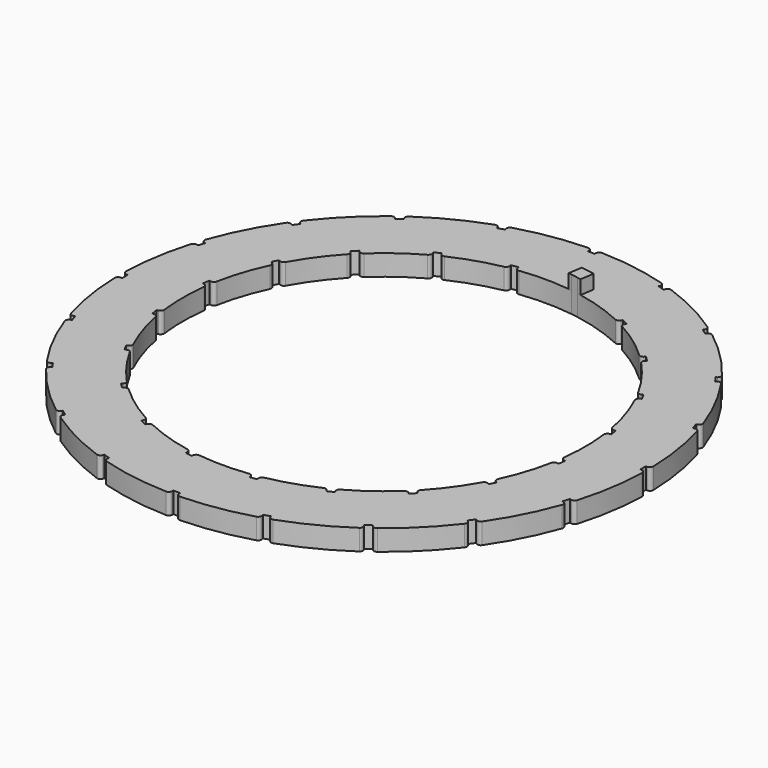
from build123d import *
from build123d import SkipClean  # not in build123d's __all__

# Parameters (mm, degrees)
F0_R     = 19
F0_R_2   = 14.5
F1_DEPTH = 1.5
F3_DEPTH = 1.501
F5_DEPTH = 1.501
F7_DEPTH = 2.5
F9_DEPTH = 1
F10_R    = 0.25
F11_R    = 0.25


with BuildPart() as f1:
    # F0 (on Top) → F1 (new body)
    with BuildSketch(Plane.XY):
        Circle(F0_R)
        Circle(F0_R_2, mode=Mode.SUBTRACT)
    extrude(amount=F1_DEPTH)

    # F2 (on face) → F3 (cut, through all)
    with BuildSketch(Plane.XY.offset(1.5)):
        with BuildLine():
            ThreePointArc((0.25, 18.998355192), (0, 19), (-0.25, 18.998355192))
            Line((-0.25, 18.998355192), (-0.25, 18.648355192))
            Line((-0.25, 18.648355192), (0.25, 18.648355192))
            Line((0.25, 18.648355192), (0.25, 18.998355192))
        make_face()
        with BuildLine():
            ThreePointArc((-5.6330504904, 18.1457637528), (-5.8713228931, 18.0700738096), (-6.1085787486, 17.9912552556))
            Line((-6.1085787486, 17.9912552556), (-6.0004228005, 17.6583854749))
            Line((-6.0004228005, 17.6583854749), (-5.5248945424, 17.8128939721))
            Line((-5.5248945424, 17.8128939721), (-5.6330504904, 18.1457637528))
        make_face()
        with BuildLine():
            ThreePointArc((-10.9646987511, 15.5169385285), (-11.1679197936, 15.3713228931), (-11.3692072482, 15.2230459024))
            Line((-11.3692072482, 15.2230459024), (-11.1634824099, 14.9398899544))
            Line((-11.1634824099, 14.9398899544), (-10.7589739128, 15.2337825805))
            Line((-10.7589739128, 15.2337825805), (-10.9646987511, 15.5169385285))
        make_face()
        with BuildLine():
            ThreePointArc((-15.2230459024, 11.3692072482), (-15.3713228931, 11.1679197936), (-15.5169385285, 10.9646987511))
            Line((-15.5169385285, 10.9646987511), (-15.2337825805, 10.7589739128))
            Line((-15.2337825805, 10.7589739128), (-14.9398899544, 11.1634824099))
            Line((-14.9398899544, 11.1634824099), (-15.2230459024, 11.3692072482))
        make_face()
        with BuildLine():
            ThreePointArc((-17.9912552556, 6.1085787486), (-18.0700738096, 5.8713228931), (-18.1457637528, 5.6330504904))
            Line((-18.1457637528, 5.6330504904), (-17.8128939721, 5.5248945424))
            Line((-17.8128939721, 5.5248945424), (-17.6583854749, 6.0004228005))
            Line((-17.6583854749, 6.0004228005), (-17.9912552556, 6.1085787486))
        make_face()
        with BuildLine():
            ThreePointArc((-18.998355192, 0.25), (-19, 0), (-18.998355192, -0.25))
            Line((-18.998355192, -0.25), (-18.648355192, -0.25))
            Line((-18.648355192, -0.25), (-18.648355192, 0.25))
            Line((-18.648355192, 0.25), (-18.998355192, 0.25))
        make_face()
        with BuildLine():
            ThreePointArc((-18.1457637528, -5.6330504904), (-18.0700738096, -5.8713228931), (-17.9912552556, -6.1085787486))
            Line((-17.9912552556, -6.1085787486), (-17.6583854749, -6.0004228005))
            Line((-17.6583854749, -6.0004228005), (-17.8128939721, -5.5248945424))
            Line((-17.8128939721, -5.5248945424), (-18.1457637528, -5.6330504904))
        make_face()
        with BuildLine():
            ThreePointArc((-15.5169385285, -10.9646987511), (-15.3713228931, -11.1679197936), (-15.2230459024, -11.3692072482))
            Line((-15.2230459024, -11.3692072482), (-14.9398899544, -11.1634824099))
            Line((-14.9398899544, -11.1634824099), (-15.2337825805, -10.7589739128))
            Line((-15.2337825805, -10.7589739128), (-15.5169385285, -10.9646987511))
        make_face()
        with BuildLine():
            ThreePointArc((-11.3692072482, -15.2230459024), (-11.1679197936, -15.3713228931), (-10.9646987511, -15.5169385285))
            Line((-10.9646987511, -15.5169385285), (-10.7589739128, -15.2337825805))
            Line((-10.7589739128, -15.2337825805), (-11.1634824099, -14.9398899544))
            Line((-11.1634824099, -14.9398899544), (-11.3692072482, -15.2230459024))
        make_face()
        with BuildLine():
            ThreePointArc((-6.1085787486, -17.9912552556), (-5.8713228931, -18.0700738096), (-5.6330504904, -18.1457637528))
            Line((-5.6330504904, -18.1457637528), (-5.5248945424, -17.8128939721))
            Line((-5.5248945424, -17.8128939721), (-6.0004228005, -17.6583854749))
            Line((-6.0004228005, -17.6583854749), (-6.1085787486, -17.9912552556))
        make_face()
        with BuildLine():
            ThreePointArc((-0.25, -18.998355192), (0, -19), (0.25, -18.998355192))
            Line((0.25, -18.998355192), (0.25, -18.648355192))
            Line((0.25, -18.648355192), (-0.25, -18.648355192))
            Line((-0.25, -18.648355192), (-0.25, -18.998355192))
        make_face()
        with BuildLine():
            ThreePointArc((5.6330504904, -18.1457637528), (5.8713228931, -18.0700738096), (6.1085787486, -17.9912552556))
            Line((6.1085787486, -17.9912552556), (6.0004228005, -17.6583854749))
            Line((6.0004228005, -17.6583854749), (5.5248945424, -17.8128939721))
            Line((5.5248945424, -17.8128939721), (5.6330504904, -18.1457637528))
        make_face()
        with BuildLine():
            ThreePointArc((10.9646987511, -15.5169385285), (11.1679197936, -15.3713228931), (11.3692072482, -15.2230459024))
            Line((11.3692072482, -15.2230459024), (11.1634824099, -14.9398899544))
            Line((11.1634824099, -14.9398899544), (10.7589739128, -15.2337825805))
            Line((10.7589739128, -15.2337825805), (10.9646987511, -15.5169385285))
        make_face()
        with BuildLine():
            ThreePointArc((15.2230459024, -11.3692072482), (15.3713228931, -11.1679197936), (15.5169385285, -10.9646987511))
            Line((15.5169385285, -10.9646987511), (15.2337825805, -10.7589739128))
            Line((15.2337825805, -10.7589739128), (14.9398899544, -11.1634824099))
            Line((14.9398899544, -11.1634824099), (15.2230459024, -11.3692072482))
        make_face()
        with BuildLine():
            ThreePointArc((17.9912552556, -6.1085787486), (18.0700738096, -5.8713228931), (18.1457637528, -5.6330504904))
            Line((18.1457637528, -5.6330504904), (17.8128939721, -5.5248945424))
            Line((17.8128939721, -5.5248945424), (17.6583854749, -6.0004228005))
            Line((17.6583854749, -6.0004228005), (17.9912552556, -6.1085787486))
        make_face()
        with BuildLine():
            ThreePointArc((18.998355192, -0.25), (19, 0), (18.998355192, 0.25))
            Line((18.998355192, 0.25), (18.648355192, 0.25))
            Line((18.648355192, 0.25), (18.648355192, -0.25))
            Line((18.648355192, -0.25), (18.998355192, -0.25))
        make_face()
        with BuildLine():
            ThreePointArc((18.1457637528, 5.6330504904), (18.0700738096, 5.8713228931), (17.9912552556, 6.1085787486))
            Line((17.9912552556, 6.1085787486), (17.6583854749, 6.0004228005))
            Line((17.6583854749, 6.0004228005), (17.8128939721, 5.5248945424))
            Line((17.8128939721, 5.5248945424), (18.1457637528, 5.6330504904))
        make_face()
        with BuildLine():
            ThreePointArc((15.5169385285, 10.9646987511), (15.3713228931, 11.1679197936), (15.2230459024, 11.3692072482))
            Line((15.2230459024, 11.3692072482), (14.9398899544, 11.1634824099))
            Line((14.9398899544, 11.1634824099), (15.2337825805, 10.7589739128))
            Line((15.2337825805, 10.7589739128), (15.5169385285, 10.9646987511))
        make_face()
        with BuildLine():
            ThreePointArc((11.3692072482, 15.2230459024), (11.1679197936, 15.3713228931), (10.9646987511, 15.5169385285))
            Line((10.9646987511, 15.5169385285), (10.7589739128, 15.2337825805))
            Line((10.7589739128, 15.2337825805), (11.1634824099, 14.9398899544))
            Line((11.1634824099, 14.9398899544), (11.3692072482, 15.2230459024))
        make_face()
        with BuildLine():
            ThreePointArc((6.1085787486, 17.9912552556), (5.8713228931, 18.0700738096), (5.6330504904, 18.1457637528))
            Line((5.6330504904, 18.1457637528), (5.5248945424, 17.8128939721))
            Line((5.5248945424, 17.8128939721), (6.0004228005, 17.6583854749))
            Line((6.0004228005, 17.6583854749), (6.1085787486, 17.9912552556))
        make_face()
    extrude(amount=-F3_DEPTH, mode=Mode.SUBTRACT)

    # F4 (on face) → F5 (cut, through all)
    with BuildSketch(Plane.XY.offset(1.5)):
        with BuildLine():
            Line((-2.5696367227, 14.6259344447), (-2.5148846599, 14.2802435255))
            ThreePointArc((-2.5148846599, 14.2802435255), (-2.2682997431, 14.3214809386), (-2.0210404896, 14.358460758))
            Line((-2.0210404896, 14.358460758), (-2.0757925524, 14.7041516772))
            Line((-2.0757925524, 14.7041516772), (-2.5696367227, 14.6259344447))
        make_face()
        with BuildLine():
            Line((-6.9635320517, 13.1160288439), (-6.8046353767, 12.8041765604))
            ThreePointArc((-6.8046353767, 12.8041765604), (-6.5828622462, 12.9195946007), (-6.3591321147, 13.0311718103))
            Line((-6.3591321147, 13.0311718103), (-6.5180287896, 13.3430240937))
            Line((-6.5180287896, 13.3430240937), (-6.9635320517, 13.1160288439))
        make_face()
        with BuildLine():
            Line((-10.6757883456, 10.322234955), (-10.4283009722, 10.0747475816))
            ThreePointArc((-10.4283009722, 10.0747475816), (-10.2530483272, 10.2530483272), (-10.0747475816, 10.4283009722))
            Line((-10.0747475816, 10.4283009722), (-10.322234955, 10.6757883456))
            Line((-10.322234955, 10.6757883456), (-10.6757883456, 10.322234955))
        make_face()
        with BuildLine():
            Line((-13.3430240937, 6.5180287896), (-13.0311718103, 6.3591321147))
            ThreePointArc((-13.0311718103, 6.3591321147), (-12.9195946007, 6.5828622462), (-12.8041765604, 6.8046353767))
            Line((-12.8041765604, 6.8046353767), (-13.1160288439, 6.9635320517))
            Line((-13.1160288439, 6.9635320517), (-13.3430240937, 6.5180287896))
        make_face()
        with BuildLine():
            Line((-14.7041516772, 2.0757925524), (-14.358460758, 2.0210404896))
            ThreePointArc((-14.358460758, 2.0210404896), (-14.3214809386, 2.2682997431), (-14.2802435255, 2.5148846599))
            Line((-14.2802435255, 2.5148846599), (-14.6259344447, 2.5696367227))
            Line((-14.6259344447, 2.5696367227), (-14.7041516772, 2.0757925524))
        make_face()
        with BuildLine():
            Line((-14.6259344447, -2.5696367227), (-14.2802435255, -2.5148846599))
            ThreePointArc((-14.2802435255, -2.5148846599), (-14.3214809386, -2.2682997431), (-14.358460758, -2.0210404896))
            Line((-14.358460758, -2.0210404896), (-14.7041516772, -2.0757925524))
            Line((-14.7041516772, -2.0757925524), (-14.6259344447, -2.5696367227))
        make_face()
        with BuildLine():
            Line((-13.1160288439, -6.9635320517), (-12.8041765604, -6.8046353767))
            ThreePointArc((-12.8041765604, -6.8046353767), (-12.9195946007, -6.5828622462), (-13.0311718103, -6.3591321147))
            Line((-13.0311718103, -6.3591321147), (-13.3430240937, -6.5180287896))
            Line((-13.3430240937, -6.5180287896), (-13.1160288439, -6.9635320517))
        make_face()
        with BuildLine():
            Line((-10.322234955, -10.6757883456), (-10.0747475816, -10.4283009722))
            ThreePointArc((-10.0747475816, -10.4283009722), (-10.2530483272, -10.2530483272), (-10.4283009722, -10.0747475816))
            Line((-10.4283009722, -10.0747475816), (-10.6757883456, -10.322234955))
            Line((-10.6757883456, -10.322234955), (-10.322234955, -10.6757883456))
        make_face()
        with BuildLine():
            Line((-6.5180287896, -13.3430240937), (-6.3591321147, -13.0311718103))
            ThreePointArc((-6.3591321147, -13.0311718103), (-6.5828622462, -12.9195946007), (-6.8046353767, -12.8041765604))
            Line((-6.8046353767, -12.8041765604), (-6.9635320517, -13.1160288439))
            Line((-6.9635320517, -13.1160288439), (-6.5180287896, -13.3430240937))
        make_face()
        with BuildLine():
            Line((-2.0757925524, -14.7041516772), (-2.0210404896, -14.358460758))
            ThreePointArc((-2.0210404896, -14.358460758), (-2.2682997431, -14.3214809386), (-2.5148846599, -14.2802435255))
            Line((-2.5148846599, -14.2802435255), (-2.5696367227, -14.6259344447))
            Line((-2.5696367227, -14.6259344447), (-2.0757925524, -14.7041516772))
        make_face()
        with BuildLine():
            Line((2.5696367227, -14.6259344447), (2.5148846599, -14.2802435255))
            ThreePointArc((2.5148846599, -14.2802435255), (2.2682997431, -14.3214809386), (2.0210404896, -14.358460758))
            Line((2.0210404896, -14.358460758), (2.0757925524, -14.7041516772))
            Line((2.0757925524, -14.7041516772), (2.5696367227, -14.6259344447))
        make_face()
        with BuildLine():
            Line((6.9635320517, -13.1160288439), (6.8046353767, -12.8041765604))
            ThreePointArc((6.8046353767, -12.8041765604), (6.5828622462, -12.9195946007), (6.3591321147, -13.0311718103))
            Line((6.3591321147, -13.0311718103), (6.5180287896, -13.3430240937))
            Line((6.5180287896, -13.3430240937), (6.9635320517, -13.1160288439))
        make_face()
        with BuildLine():
            Line((10.6757883456, -10.322234955), (10.4283009722, -10.0747475816))
            ThreePointArc((10.4283009722, -10.0747475816), (10.2530483272, -10.2530483272), (10.0747475816, -10.4283009722))
            Line((10.0747475816, -10.4283009722), (10.322234955, -10.6757883456))
            Line((10.322234955, -10.6757883456), (10.6757883456, -10.322234955))
        make_face()
        with BuildLine():
            Line((13.3430240937, -6.5180287896), (13.0311718103, -6.3591321147))
            ThreePointArc((13.0311718103, -6.3591321147), (12.9195946007, -6.5828622462), (12.8041765604, -6.8046353767))
            Line((12.8041765604, -6.8046353767), (13.1160288439, -6.9635320517))
            Line((13.1160288439, -6.9635320517), (13.3430240937, -6.5180287896))
        make_face()
        with BuildLine():
            Line((14.7041516772, -2.0757925524), (14.358460758, -2.0210404896))
            ThreePointArc((14.358460758, -2.0210404896), (14.3214809386, -2.2682997431), (14.2802435255, -2.5148846599))
            Line((14.2802435255, -2.5148846599), (14.6259344447, -2.5696367227))
            Line((14.6259344447, -2.5696367227), (14.7041516772, -2.0757925524))
        make_face()
        with BuildLine():
            Line((14.6259344447, 2.5696367227), (14.2802435255, 2.5148846599))
            ThreePointArc((14.2802435255, 2.5148846599), (14.3214809386, 2.2682997431), (14.358460758, 2.0210404896))
            Line((14.358460758, 2.0210404896), (14.7041516772, 2.0757925524))
            Line((14.7041516772, 2.0757925524), (14.6259344447, 2.5696367227))
        make_face()
        with BuildLine():
            Line((13.1160288439, 6.9635320517), (12.8041765604, 6.8046353767))
            ThreePointArc((12.8041765604, 6.8046353767), (12.9195946007, 6.5828622462), (13.0311718103, 6.3591321147))
            Line((13.0311718103, 6.3591321147), (13.3430240937, 6.5180287896))
            Line((13.3430240937, 6.5180287896), (13.1160288439, 6.9635320517))
        make_face()
        with BuildLine():
            Line((10.322234955, 10.6757883456), (10.0747475816, 10.4283009722))
            ThreePointArc((10.0747475816, 10.4283009722), (10.2530483272, 10.2530483272), (10.4283009722, 10.0747475816))
            Line((10.4283009722, 10.0747475816), (10.6757883456, 10.322234955))
            Line((10.6757883456, 10.322234955), (10.322234955, 10.6757883456))
        make_face()
        with BuildLine():
            Line((6.5180287896, 13.3430240937), (6.3591321147, 13.0311718103))
            ThreePointArc((6.3591321147, 13.0311718103), (6.5828622462, 12.9195946007), (6.8046353767, 12.8041765604))
            Line((6.8046353767, 12.8041765604), (6.9635320517, 13.1160288439))
            Line((6.9635320517, 13.1160288439), (6.5180287896, 13.3430240937))
        make_face()
        with BuildLine():
            Line((2.0757925524, 14.7041516772), (2.0210404896, 14.358460758))
            ThreePointArc((2.0210404896, 14.358460758), (2.2682997431, 14.3214809386), (2.5148846599, 14.2802435255))
            Line((2.5148846599, 14.2802435255), (2.5696367227, 14.6259344447))
            Line((2.5696367227, 14.6259344447), (2.0757925524, 14.7041516772))
        make_face()
    extrude(amount=-F5_DEPTH, mode=Mode.SUBTRACT)

    # F6 (on face) → F7 (join)
    with BuildSketch(Plane(origin=(0, 0, 0), x_dir=(1, 0, 0), z_dir=(0, 0, -1))):
        with BuildLine():
            Line((2.5696367227, -14.6259344447), (2.5148846599, -14.2802435255))
            ThreePointArc((2.5148846599, -14.2802435255), (2.2682997431, -14.3214809386), (2.0210404896, -14.358460758))
            Line((2.0210404896, -14.358460758), (2.0757925524, -14.7041516772))
            Line((2.0757925524, -14.7041516772), (2.5696367227, -14.6259344447))
        make_face()
    extrude(amount=-F7_DEPTH)

    # F8 (on face) → F9 (join, through all)
    with BuildSketch(Plane.XY.offset(1.5)):
        with BuildLine():
            Line((1.9295410637, 15.3788694245), (1.7731065987, 14.3911810839))
            ThreePointArc((1.7731065987, 14.3911810839), (2.2682997431, 14.3214809386), (2.7607949393, 14.2347466189))
            Line((2.7607949393, 14.2347466189), (2.9172294043, 15.2224349595))
            Line((2.9172294043, 15.2224349595), (1.9295410637, 15.3788694245))
        make_face()
    with SkipClean():  # cleaning this boolean's faces spoils the solid; the shape is the same uncleaned
        extrude(amount=F9_DEPTH)

    # F10
    f10_edges = [f1.edges().sort_by_distance(p)[0] for p in [
        (6.108579, 17.991255, 0.75),
        (5.63305, 18.145764, 0.75),
        (0.25, 18.998355, 0.75),
        (-0.25, 18.998355, 0.75),
        (-5.63305, 18.145764, 0.75),
        (-6.108579, 17.991255, 0.75),
        (10.964699, 15.516939, 0.75),
        (11.369207, 15.223046, 0.75),
        (15.223046, 11.369207, 0.75),
        (15.516939, 10.964699, 0.75),
        (17.991255, 6.108579, 0.75),
        (18.145764, 5.63305, 0.75),
        (18.998355, 0.25, 0.75),
        (18.998355, -0.25, 0.75),
        (18.145764, -5.63305, 0.75),
        (17.991255, -6.108579, 0.75),
        (15.516939, -10.964699, 0.75),
        (15.223046, -11.369207, 0.75),
        (11.369207, -15.223046, 0.75),
        (10.964699, -15.516939, 0.75),
        (6.108579, -17.991255, 0.75),
        (5.63305, -18.145764, 0.75),
        (0.25, -18.998355, 0.75),
        (-0.25, -18.998355, 0.75),
        (-5.63305, -18.145764, 0.75),
        (-6.108579, -17.991255, 0.75),
        (-10.964699, -15.516939, 0.75),
        (-11.369207, -15.223046, 0.75),
        (-15.223046, -11.369207, 0.75),
        (-15.516939, -10.964699, 0.75),
        (-17.991255, -6.108579, 0.75),
        (-18.145764, -5.63305, 0.75),
        (-18.998355, -0.25, 0.75),
        (-18.998355, 0.25, 0.75),
        (-18.145764, 5.63305, 0.75),
        (-17.991255, 6.108579, 0.75),
        (-15.516939, 10.964699, 0.75),
        (-15.223046, 11.369207, 0.75),
        (-11.369207, 15.223046, 0.75),
        (-10.964699, 15.516939, 0.75),
    ]]
    fillet(f10_edges, radius=F10_R)

    # F11
    f11_edges = [f1.edges().sort_by_distance(p)[0] for p in [
        (-12.804177, -6.804635, 0.75),
        (-13.031172, -6.359132, 0.75),
        (-14.280244, -2.514885, 0.75),
        (-14.358461, -2.02104, 0.75),
        (-10.428301, -10.074748, 0.75),
        (-10.074748, -10.428301, 0.75),
        (-14.358461, 2.02104, 0.75),
        (-14.280244, 2.514885, 0.75),
        (-13.031172, 6.359132, 0.75),
        (-12.804177, 6.804635, 0.75),
        (-10.428301, 10.074748, 0.75),
        (-10.074748, 10.428301, 0.75),
        (-6.804635, 12.804177, 0.75),
        (-6.359132, 13.031172, 0.75),
        (-2.514885, 14.280244, 0.75),
        (-2.02104, 14.358461, 0.75),
        (6.359132, 13.031172, 0.75),
        (6.804635, 12.804177, 0.75),
        (10.074748, 10.428301, 0.75),
        (10.428301, 10.074748, 0.75),
        (12.804177, 6.804635, 0.75),
        (13.031172, 6.359132, 0.75),
        (14.280244, 2.514885, 0.75),
        (14.358461, 2.02104, 0.75),
        (14.358461, -2.02104, 0.75),
        (14.280244, -2.514885, 0.75),
        (13.031172, -6.359132, 0.75),
        (12.804177, -6.804635, 0.75),
        (10.428301, -10.074748, 0.75),
        (10.074748, -10.428301, 0.75),
        (6.804635, -12.804177, 0.75),
        (6.359132, -13.031172, 0.75),
        (2.514885, -14.280244, 0.75),
        (2.02104, -14.358461, 0.75),
        (-2.02104, -14.358461, 0.75),
        (-2.514885, -14.280244, 0.75),
        (-6.359132, -13.031172, 0.75),
        (-6.804635, -12.804177, 0.75),
    ]]
    fillet(f11_edges, radius=F11_R)


solid = f1.part
